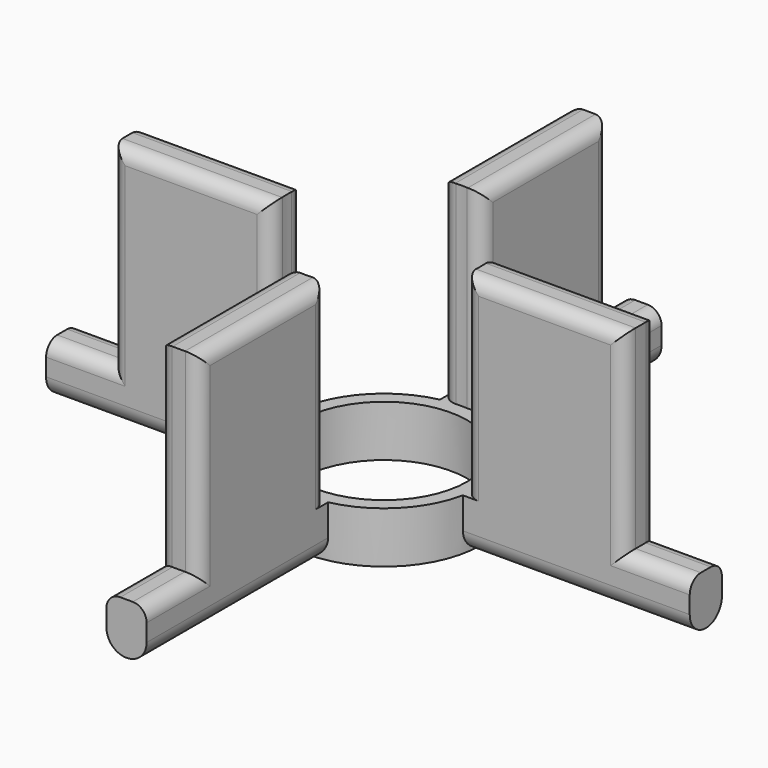
from build123d import *

# Parameters (mm, degrees)
F0_R     = 6
F1_DEPTH = 3.7
F2_R     = 1.44999
F4_DEPTH = 14
F5_R     = 1


# Not quite as in the source:
# - a fillet or chamfer is up to 0.001 mm smaller than in the source, because OpenCascade refuses the exact size


with BuildPart() as f1:
    # F0 (on Top) → F1 (new body)
    with BuildSketch(Plane.XY):
        with BuildLine():
            ThreePointArc((6.8481749394, -1.45), (6.9619402675, -0.7289634506), (7, 0))
            ThreePointArc((7, 0), (6.9619402675, 0.7289634506), (6.8481749394, 1.45))
            ThreePointArc((6.8481749394, 1.45), (4.9497474683, 4.9497474683), (1.45, 6.8481749394))
            ThreePointArc((1.45, 6.8481749394), (0.7289634506, 6.9619402675), (0, 7))
            ThreePointArc((0, 7), (-0.7289634506, 6.9619402675), (-1.45, 6.8481749394))
            ThreePointArc((-1.45, 6.8481749394), (-4.9497474683, 4.9497474683), (-6.8481749394, 1.45))
            ThreePointArc((-6.8481749394, 1.45), (-6.9619402675, 0.7289634506), (-7, 0))
            ThreePointArc((-7, 0), (-6.9619402675, -0.7289634506), (-6.8481749394, -1.45))
            ThreePointArc((-6.8481749394, -1.45), (-4.9497474683, -4.9497474683), (-1.45, -6.8481749394))
            ThreePointArc((-1.45, -6.8481749394), (-0.7289634506, -6.9619402675), (0, -7))
            ThreePointArc((0, -7), (0.7289634506, -6.9619402675), (1.45, -6.8481749394))
            ThreePointArc((1.45, -6.8481749394), (4.9497474683, -4.9497474683), (6.8481749394, -1.45))
        make_face()
        Circle(F0_R, mode=Mode.SUBTRACT)
        with BuildLine():
            Line((23.2, 0), (7, 0))
            ThreePointArc((7, 0), (6.9619402675, -0.7289634506), (6.8481749394, -1.45))
            Line((6.8481749394, -1.45), (23.2, -1.45))
            Line((23.2, -1.45), (23.2, 0))
        make_face()
        with BuildLine():
            ThreePointArc((6.8481749394, 1.45), (6.9619402675, 0.7289634506), (7, 0))
            Line((7, 0), (23.2, 0))
            Line((23.2, 0), (23.2, 1.45))
            Line((23.2, 1.45), (6.8481749394, 1.45))
        make_face()
        with BuildLine():
            ThreePointArc((0, 7), (0.7289634506, 6.9619402675), (1.45, 6.8481749394))
            Line((1.45, 6.8481749394), (1.45, 23.2))
            Line((1.45, 23.2), (0, 23.2))
            Line((0, 23.2), (0, 7))
        make_face()
        with BuildLine():
            Line((1.45, -23.2), (1.45, -6.8481749394))
            ThreePointArc((1.45, -6.8481749394), (0.7289634506, -6.9619402675), (0, -7))
            Line((0, -7), (0, -23.2))
            Line((0, -23.2), (1.45, -23.2))
        make_face()
        with BuildLine():
            ThreePointArc((-1.45, 6.8481749394), (-0.7289634506, 6.9619402675), (0, 7))
            Line((0, 7), (0, 23.2))
            Line((0, 23.2), (-1.45, 23.2))
            Line((-1.45, 23.2), (-1.45, 6.8481749394))
        make_face()
        with BuildLine():
            Line((0, -23.2), (0, -7))
            ThreePointArc((0, -7), (-0.7289634506, -6.9619402675), (-1.45, -6.8481749394))
            Line((-1.45, -6.8481749394), (-1.45, -23.2))
            Line((-1.45, -23.2), (0, -23.2))
        make_face()
        with BuildLine():
            ThreePointArc((-7, 0), (-6.9619402675, 0.7289634506), (-6.8481749394, 1.45))
            Line((-6.8481749394, 1.45), (-23.2, 1.45))
            Line((-23.2, 1.45), (-23.2, 0))
            Line((-23.2, 0), (-7, 0))
        make_face()
        with BuildLine():
            Line((-23.2, -1.45), (-6.8481749394, -1.45))
            ThreePointArc((-6.8481749394, -1.45), (-6.9619402675, -0.7289634506), (-7, 0))
            Line((-7, 0), (-23.2, 0))
            Line((-23.2, 0), (-23.2, -1.45))
        make_face()
    extrude(amount=F1_DEPTH)

    # F2 (radius 1.45 in the source; OpenCascade refuses exactly that, so slightly less here)
    f2_edges = [f1.edges().sort_by_distance(p)[0] for p in [
        (1.45, 15.024087, 0),
        (15.024087, 1.45, 0),
        (15.024087, -1.45, 0),
        (1.45, -15.024087, 0),
        (-1.45, -15.024087, 0),
        (-15.024087, -1.45, 0),
        (-15.024087, 1.45, 0),
        (-1.45, 15.024087, 0),
    ]]
    fillet(f2_edges, radius=F2_R)

    # F3 (on face) → F4 (join)
    with BuildSketch(Plane.XY.offset(3.7)):
        with BuildLine():
            Line((18.4430881362, 1.45), (18.4430881362, -1.45))
            ThreePointArc((18.4430881362, -1.45), (18.5, 0), (18.4430881362, 1.45))
        make_face()
        with BuildLine():
            Line((6.8481749394, -1.45), (18.4430881362, -1.45))
            Line((18.4430881362, -1.45), (18.4430881362, 1.45))
            Line((18.4430881362, 1.45), (6.8481749394, 1.45))
            ThreePointArc((6.8481749394, 1.45), (7, 0), (6.8481749394, -1.45))
        make_face()
        with BuildLine():
            ThreePointArc((-18.4430881362, 1.45), (-18.5, 0), (-18.4430881362, -1.45))
            Line((-18.4430881362, -1.45), (-18.4430881362, 1.45))
        make_face()
        with BuildLine():
            Line((-18.4430881362, 1.45), (-18.4430881362, -1.45))
            Line((-18.4430881362, -1.45), (-6.8481749394, -1.45))
            ThreePointArc((-6.8481749394, -1.45), (-7, 0), (-6.8481749394, 1.45))
            Line((-6.8481749394, 1.45), (-18.4430881362, 1.45))
        make_face()
        with BuildLine():
            ThreePointArc((-1.45, -18.4430881362), (0, -18.5), (1.45, -18.4430881362))
            Line((1.45, -18.4430881362), (-1.45, -18.4430881362))
        make_face()
        with BuildLine():
            Line((-1.45, -18.4430881362), (1.45, -18.4430881362))
            Line((1.45, -18.4430881362), (1.45, -6.8481749394))
            ThreePointArc((1.45, -6.8481749394), (0, -7), (-1.45, -6.8481749394))
            Line((-1.45, -6.8481749394), (-1.45, -18.4430881362))
        make_face()
        with BuildLine():
            Line((1.45, 6.8481749394), (1.45, 18.4430881362))
            Line((1.45, 18.4430881362), (-1.45, 18.4430881362))
            Line((-1.45, 18.4430881362), (-1.45, 6.8481749394))
            ThreePointArc((-1.45, 6.8481749394), (0, 7), (1.45, 6.8481749394))
        make_face()
        with BuildLine():
            Line((-1.45, 18.4430881362), (1.45, 18.4430881362))
            ThreePointArc((1.45, 18.4430881362), (0, 18.5), (-1.45, 18.4430881362))
        make_face()
    extrude(amount=F4_DEPTH)

    # F5
    f5_edges = [f1.edges().sort_by_distance(p)[0] for p in [
        (12.645632, 1.45, 17.7),
        (18.443088, 1.45, 10.7),
        (20.821544, 1.45, 3.7),
        (20.821544, -1.45, 3.7),
        (18.443088, -1.45, 10.7),
        (12.645632, -1.45, 17.7),
        (1.45, 12.645632, 17.7),
        (-1.45, 12.645632, 17.7),
        (1.45, 18.443088, 10.7),
        (-1.45, 18.443088, 10.7),
        (1.45, 20.821544, 3.7),
        (-1.45, 20.821544, 3.7),
        (0, 18.5, 3.7),
        (-18.443088, 1.45, 10.7),
        (-18.443088, -1.45, 10.7),
        (-20.821544, 1.45, 3.7),
        (-1.45, -18.443088, 10.7),
        (1.45, -18.443088, 10.7),
        (-1.45, -20.821544, 3.7),
        (1.45, -20.821544, 3.7),
        (-20.821544, -1.45, 3.7),
        (-12.645632, 1.45, 17.7),
        (-12.645632, -1.45, 17.7),
        (-1.45, -12.645632, 17.7),
        (1.45, -12.645632, 17.7),
        (-1.45, -6.848175, 10.7),
        (1.45, -6.848175, 10.7),
        (6.848175, -1.45, 10.7),
        (6.848175, 1.45, 10.7),
        (1.45, 6.848175, 10.7),
        (-1.45, 6.848175, 10.7),
        (-6.848175, 1.45, 10.7),
        (-6.848175, -1.45, 10.7),
    ]]
    fillet(f5_edges, radius=F5_R)


solid = f1.part
